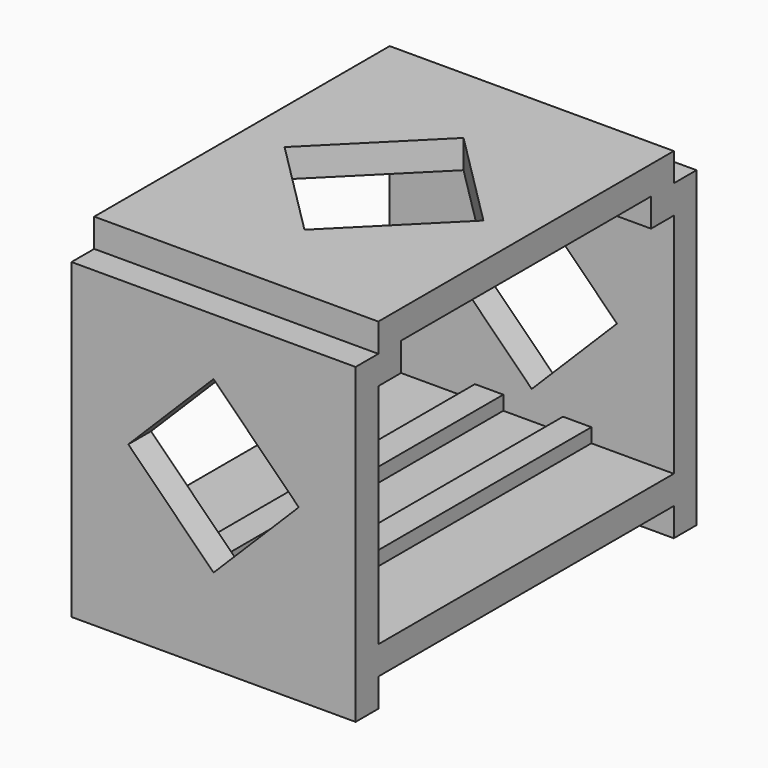
from build123d import *

# Parameters (mm, degrees)
F1_DEPTH = 20
F2_T     = -2
F3_W     = 2
F3_H     = 1
F4_DEPTH = 26
F6_DEPTH = 30.001
F8_DEPTH = 2


# Not quite as in the source:
# - a shell that OpenCascade refuses in one call is made with other operations: the cavity is built on its own and cut out


with BuildPart() as f1:
    # F0 (on Right) → F1 (new body)
    with BuildSketch(Plane.YZ):
        Polygon((-13, -2), (-13, 0), (13, 0), (13, -2), (15, -2), (15, 20), (13, 20), (13, 22), (-13, 22), (-13, 20), (-15, 20), (-15, -2), align=None)
    extrude(amount=F1_DEPTH)

    # F2: a shell. OpenCascade refuses it in one call, so the cavity is built on its own and cut out:
    # the body offset inwards by the wall thickness, plus a prism from it out through each open face.
    f2_core = offset(f1.part, amount=F2_T, kind=Kind.INTERSECTION, mode=Mode.PRIVATE)
    f2_exits = [f2_core.faces().sort_by_distance(p)[0] for p in [
        (2, 0, 10.86087),
        (18, 0, 10.86087),
    ]]
    add(f2_core, mode=Mode.SUBTRACT)
    extrude(f2_exits, amount=-F2_T, mode=Mode.SUBTRACT)

    # F3 (on face) → F4 (join, through all)
    with BuildSketch(Plane.XZ.offset(-13)):
        with Locations((7, 2.5)):
            Rectangle(F3_W, F3_H)
        with Locations((13.2, 2.5)):
            Rectangle(F3_W, F3_H)
    extrude(amount=F4_DEPTH)

    # F5 (on face) → F6 (cut, through all)
    with BuildSketch(Plane.XZ.offset(15)):
        Polygon((16, 10), (10, 16), (4, 10), (10, 4), align=None)
    extrude(amount=-F6_DEPTH, mode=Mode.SUBTRACT)

    # F7 (on face) → F8 (cut, through all)
    with BuildSketch(Plane.XY.offset(22)):
        Polygon((17, 0), (10, 7), (3, 0), (10, -7), align=None)
    extrude(amount=-F8_DEPTH, mode=Mode.SUBTRACT)


solid = f1.part
